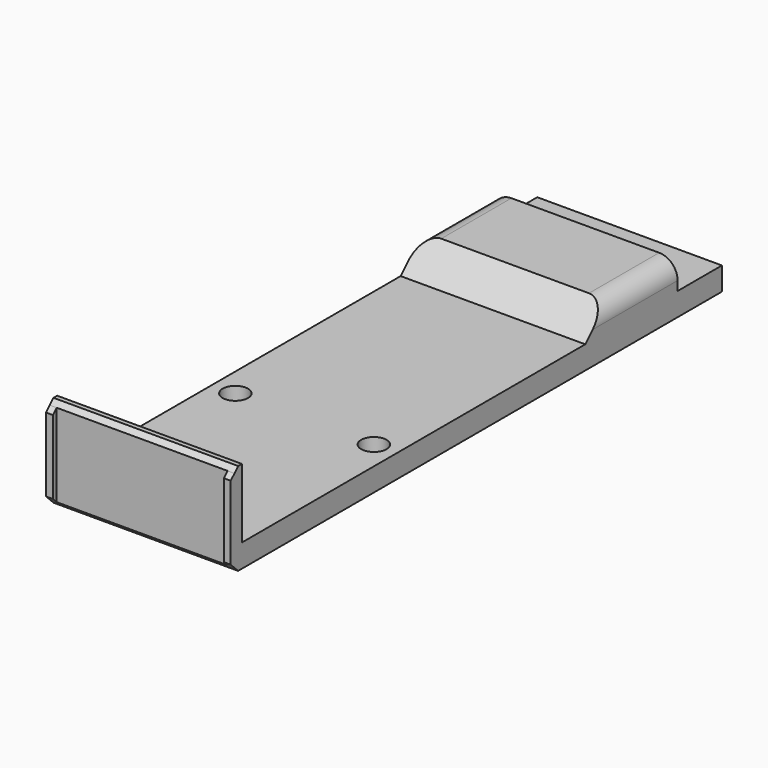
from build123d import *

# Parameters (mm, degrees)
F0_W      = 40
F0_H      = 131.9999998143
F1_DEPTH  = 5
F2_W      = 40
F2_H      = 2
F3_DEPTH  = 15
F4_D      = 5.5
F4_DEPTH  = 8
F4_TIP    = 1.6523667023
F5_SIZE   = 1
F6_W      = 40
F6_H      = 25
F7_DEPTH  = 6
F8_R      = 2
F9_DEPTH  = 5
F10_SIZE  = 5.99999
F11_R     = 4
F12_D     = 2.8
F12_DEPTH = 8
F12_TIP   = 0.8412048666
F13_W     = 1.5
F13_H     = 18
F14_DEPTH = 1
F15_SIZE  = 0.99999


# Not quite as in the source:
# - a fillet or chamfer is up to 0.001 mm smaller than in the source, because OpenCascade refuses the exact size


with BuildPart() as f1:
    # F0 (on Top) → F1 (new body)
    with BuildSketch(Plane.XY):
        with Locations((0, 9.28e-08)):
            Rectangle(F0_W, F0_H)
    extrude(amount=F1_DEPTH)

    # F2 (on face) → F3 (join)
    with BuildSketch(Plane.XY.offset(5)):
        with Locations((0, -64.9999998143)):
            Rectangle(F2_W, F2_H)
    extrude(amount=F3_DEPTH)

    # F4
    with Locations(Plane.XY.offset(5)):
        with Locations((-15, -21.9999998143), (15, -21.9999998143)):
            Hole(F4_D / 2, depth=F4_DEPTH)
            with Locations((0, 0, -(F4_DEPTH + F4_TIP / 2))):  # 118° drill point
                Cone(0, F4_D / 2, F4_TIP, mode=Mode.SUBTRACT)

    # F5
    f5_edges = [f1.edges().sort_by_distance(p)[0] for p in [
        (0, -66, 20),
        (0, -66, 0),
        (-17.75, -22, 0),
        (12.25, -22, 0),
    ]]
    chamfer(f5_edges, length=F5_SIZE)

    # F6 (on face) → F7 (join)
    with BuildSketch(Plane.XY.offset(5)):
        with Locations((0, 41.5)):
            Rectangle(F6_W, F6_H)
    extrude(amount=F7_DEPTH)

    # F8 (on face) → F9 (cut)
    with BuildSketch(Plane(origin=(0, 54, 0), x_dir=(-1, 0, 0), z_dir=(0, 1, 0))):
        with Locations((-15, 7.5)):
            Circle(F8_R)
        with Locations((15, 7.5)):
            Circle(F8_R)
    extrude(amount=-F9_DEPTH, mode=Mode.SUBTRACT)

    # F10 (size 6 in the source; OpenCascade refuses exactly that, so slightly less here)
    f10_edges = [f1.edges().sort_by_distance(p)[0] for p in [
        (0, 29, 11),
    ]]
    chamfer(f10_edges, length=F10_SIZE)

    # F11
    f11_edges = [f1.edges().sort_by_distance(p)[0] for p in [
        (-20, 44.499995, 11),
        (20, 44.499995, 11),
    ]]
    fillet(f11_edges, radius=F11_R)

    # F12
    with Locations(Plane.XY.offset(5)):
        with Locations((10, 61), (-10, 61)):
            Hole(F12_D / 2, depth=F12_DEPTH)
            with Locations((0, 0, -(F12_DEPTH + F12_TIP / 2))):  # 118° drill point
                Cone(0, F12_D / 2, F12_TIP, mode=Mode.SUBTRACT)

    # F13 (on face) → F14 (join)
    with BuildSketch(Plane.XZ.offset(65.9999998143)):
        with Locations((-19.25, 10)):
            Rectangle(F13_W, F13_H)
        with Locations((19.25, 10)):
            Rectangle(F13_W, F13_H)
    extrude(amount=F14_DEPTH)

    # F15 (size 1 in the source; OpenCascade refuses exactly that, so slightly less here)
    f15_edges = [f1.edges().sort_by_distance(p)[0] for p in [
        (-19.25, -67, 19),
        (-19.25, -67, 1),
        (19.25, -67, 19),
        (19.25, -67, 1),
    ]]
    chamfer(f15_edges, length=F15_SIZE)


solid = f1.part
